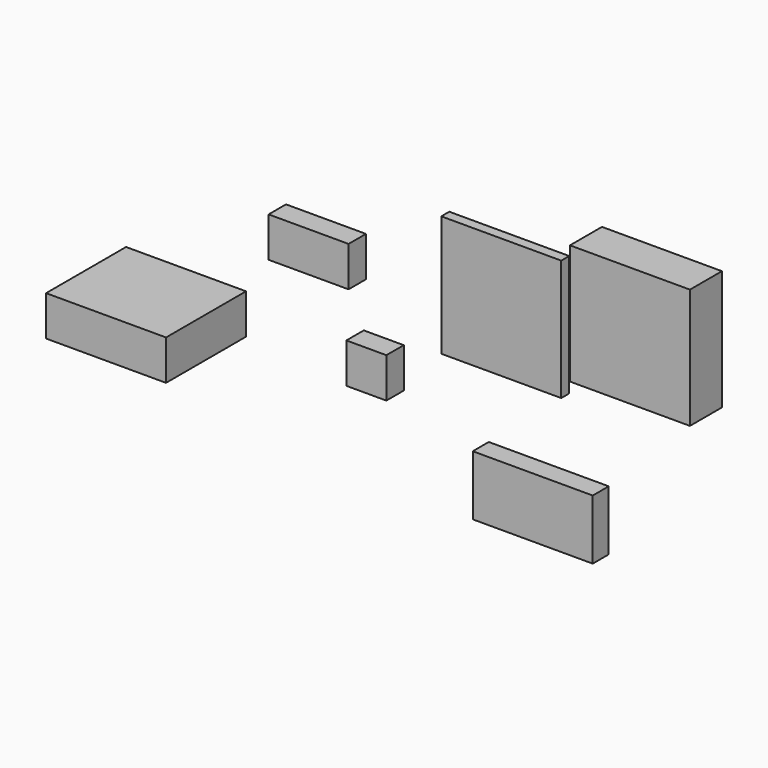
from build123d import *

# Parameters (mm, degrees)
F1_DEPTH  = 60.325
F2_SIZE   = 5.08
F3_W      = 304.8
F3_H      = 307.4512779713
F4_DEPTH  = 25.4
F5_W      = 304.8
F5_H      = 304.8
F6_DEPTH  = 101.6
F7_W      = 101.6
F7_H      = 101.6
F8_DEPTH  = 60.325
F9_SIZE   = 5.08
F10_W     = 304.8
F10_H     = 152.4
F11_DEPTH = 50.8
F12_W     = 304.8
F12_H     = 101.6
F13_DEPTH = 254


with BuildPart() as f1:
    # F0 (on Front) → F1 (new body)
    with BuildSketch(Plane.XZ):
        Polygon((-34.8327495575, 40.6072164297), (-238.0327495575, 40.6072164297), (-238.0327495575, -60.9927835703), (-135.3522986174, -60.9927835703), (-34.8327495575, -60.9927835703), align=None)
    extrude(amount=F1_DEPTH)

    # F2
    f2_edges = [f1.edges().sort_by_distance(p)[0] for p in [
        (-136.43275, 0, -60.992784),
        (-136.43275, 0, 40.607216),
        (-34.83275, 0, -10.192784),
    ]]
    chamfer(f2_edges, length=F2_SIZE)


with BuildPart() as f4:
    # F3 (on Front) → F4 (new body)
    with BuildSketch(Plane.XZ):
        with Locations((325.1804988623, 1.9569396973)):
            Rectangle(F3_W, F3_H)
    extrude(amount=F4_DEPTH)


with BuildPart() as f6:
    # F5 (on Front) → F6 (new body)
    with BuildSketch(Plane.XZ):
        with Locations((713.1468355656, 95.5299821684)):
            Rectangle(F5_W, F5_H)
    extrude(amount=F6_DEPTH)


with BuildPart() as f8:
    # F7 (on Front) → F8 (new body)
    with BuildSketch(Plane.XZ):
        with Locations((10.3937499225, -227.8598965335)):
            Rectangle(F7_W, F7_H)
    extrude(amount=F8_DEPTH)

    # F9
    f9_edges = [f8.edges().sort_by_distance(p)[0] for p in [
        (61.19375, 0, -227.859897),
        (10.39375, 0, -278.659897),
        (-40.40625, 0, -227.859897),
        (10.39375, 0, -177.059897),
    ]]
    chamfer(f9_edges, length=F9_SIZE)


with BuildPart() as f11:
    # F10 (on Front) → F11 (new body)
    with BuildSketch(Plane.XZ):
        with Locations((425.5021352335, -402.9936790466)):
            Rectangle(F10_W, F10_H)
    extrude(amount=F11_DEPTH)


with BuildPart() as f13:
    # F12 (on Front) → F13 (new body)
    with BuildSketch(Plane.XZ):
        with Locations((-496.0762047155, -241.1027252674)):
            Rectangle(F12_W, F12_H)
    extrude(amount=F13_DEPTH)


solid = Compound([f1.part, f4.part, f6.part, f8.part, f11.part, f13.part])
